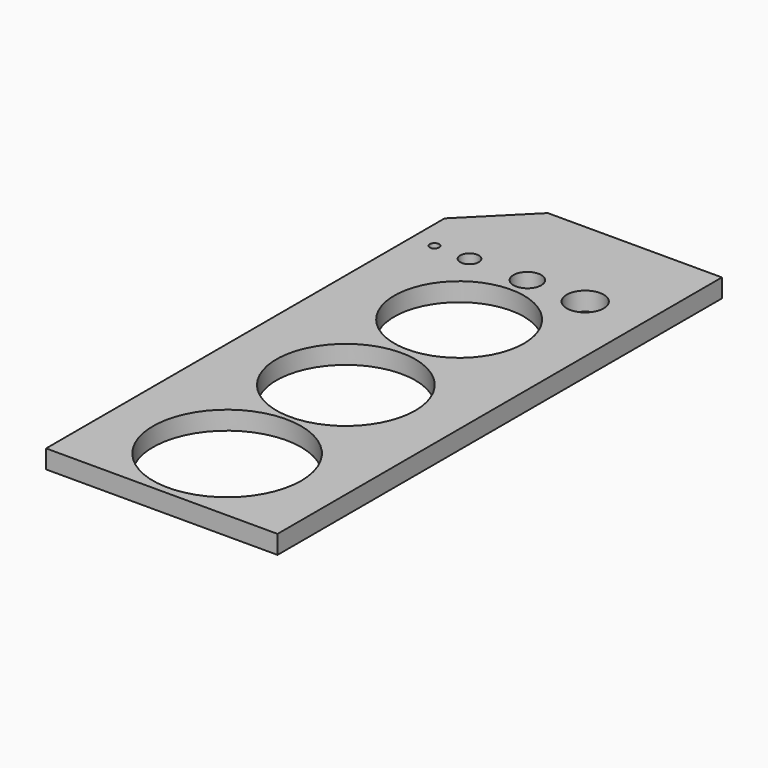
from build123d import *

# Parameters (mm, degrees)
F1_DEPTH = 2
F2_SIZE  = 1.99999
F3_R     = 1
F3_R_2   = 0.5
F3_R_3   = 1.5
F3_R_4   = 2
F4_DEPTH = 25.4
F5_R     = 7.5
F5_R_2   = 8
F5_R_3   = 7
F6_DEPTH = 25.4


# Not quite as in the source:
# - a fillet or chamfer is up to 0.001 mm smaller than in the source, because OpenCascade refuses the exact size


with BuildPart() as f1:
    # F0 (on Top) → F1 (new body)
    with BuildSketch(Plane.XY):
        Polygon((-12.5, -30), (12.5, -30), (12.5, 30), (-9.1340300441, 30), (-12.5, 26.6340300441), align=None)
    extrude(amount=F1_DEPTH)

    # F2 (size 2 in the source; OpenCascade refuses exactly that, so slightly less here)
    f2_edges = [f1.edges().sort_by_distance(p)[0] for p in [
        (-10.817015, 28.317015, 2),
    ]]
    chamfer(f2_edges, length=F2_SIZE)

    # F3 (on face) → F4 (cut)
    with BuildSketch(Plane.XY.offset(2)):
        with Locations((-6.25, 19.3575184322)):
            Circle(F3_R)
        with Locations((-10.0335823372, 19.3575184322)):
            Circle(F3_R_2)
        with Locations((0, 19.3575184322)):
            Circle(F3_R_3)
        with Locations((6.25, 19.3575184322)):
            Circle(F3_R_4)
    extrude(amount=-F4_DEPTH, mode=Mode.SUBTRACT)

    # F5 (on face) → F6 (cut)
    with BuildSketch(Plane.XY.offset(2)):
        with Locations((0, -5.1503664152)):
            Circle(F5_R)
        with Locations((0, -21.1835757454)):
            Circle(F5_R_2)
        with Locations((0, 10.1449948387)):
            Circle(F5_R_3)
    extrude(amount=-F6_DEPTH, mode=Mode.SUBTRACT)


solid = f1.part
